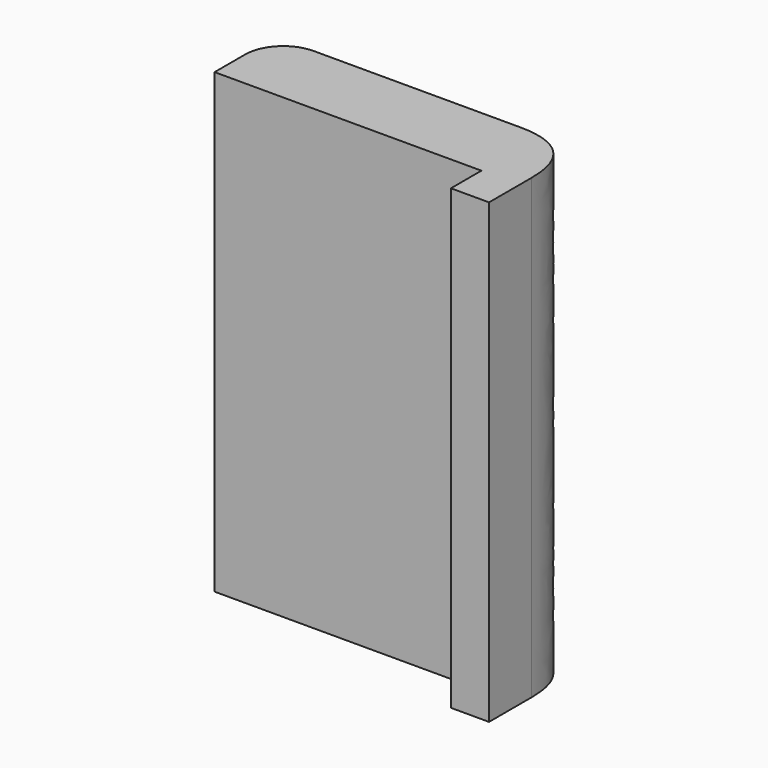
from build123d import *

# Parameters (mm, degrees)
F0_W        = 40
F0_H        = 15
F1_DEPTH    = 60
F2_W        = 35
F2_H        = 5
F3_DEPTH    = 60
F4_T1_DEPTH = 100
F5_R        = 5


# Not quite as in the source:
# - a fillet or chamfer that OpenCascade refuses, or shapes differently, is made with other operations: its cross-section is extruded or revolved along the edge and cut away or added


with BuildPart() as f1:
    # F0 (on Top) → F1 (new body)
    with BuildSketch(Plane.XY):
        with Locations((20, -7.5)):
            Rectangle(F0_W, F0_H)
    extrude(amount=F1_DEPTH)

    # F2 (on face) → F3 (cut, through all)
    with BuildSketch(Plane.XY.offset(60)):
        with Locations((17.5, -12.5)):
            Rectangle(F2_W, F2_H)
    extrude(amount=-F3_DEPTH, mode=Mode.SUBTRACT)

    # F4: fillet of radius 8 on 1 edges, made by hand

    # F4_s2 → F4_t1 (cut)
    with BuildSketch(Plane.XY.offset(-20)):
        with BuildLine():
            add(Edge.make_bspline(
                [(32, 0), (40, 0), (40, -8)],
                knots=[0, 0, 0, 1, 1, 1], degree=2, weights=[1, 1, 1]))
            Line((40, -8), (40, 0))
            Line((40, 0), (32, 0))
        make_face()
    extrude(amount=F4_T1_DEPTH, mode=Mode.SUBTRACT)

    # F5
    f5_edges = [f1.edges().sort_by_distance(p)[0] for p in [
        (0, 0, 30),
    ]]
    fillet(f5_edges, radius=F5_R)


solid = f1.part
